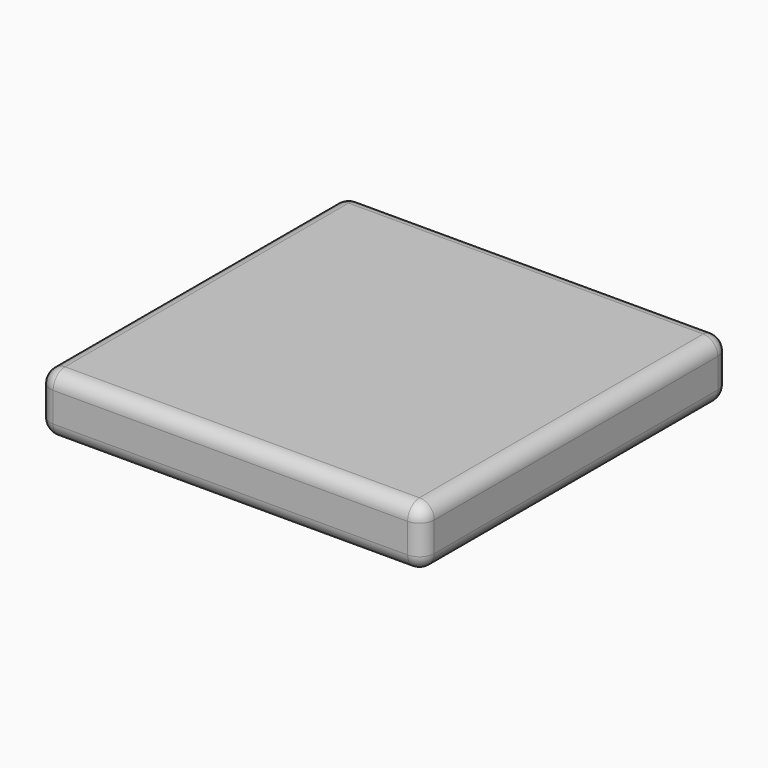
from build123d import *

# Parameters (mm, degrees)
F0_W         = 520
F0_H         = 520
F1_DEPTH     = 80
F2_R         = 20
F3_T1_DEPTH  = 40
F3_S5_W      = 20
F3_S5_H      = 20
F3_T6_DEPTH  = 20
F3_S11_W     = 20
F3_S11_H     = 20
F3_T12_DEPTH = 20
F3_S17_W     = 20
F3_S17_H     = 20
F3_T18_DEPTH = 20
F3_S23_W     = 20
F3_S23_H     = 20
F3_T24_DEPTH = 20
F3_S29_W     = 20
F3_S29_H     = 20
F3_T30_DEPTH = 20
F3_S35_W     = 20
F3_S35_H     = 20
F3_T36_DEPTH = 20
F3_S41_W     = 20
F3_S41_H     = 20
F3_T42_DEPTH = 20
F3_S47_W     = 20
F3_S47_H     = 20
F3_T48_DEPTH = 20


# Not quite as in the source:
# - a fillet or chamfer that OpenCascade refuses, or shapes differently, is made with other operations: its cross-section is extruded or revolved along the edge and cut away or added


with BuildPart() as f1:
    # F0 (on Top) → F1 (new body)
    with BuildSketch(Plane.XY):
        Rectangle(F0_W, F0_H)
    extrude(amount=F1_DEPTH)

    # F2
    f2_edges = [f1.edges().sort_by_distance(p)[0] for p in [
        (260, 0, 80),
        (0, 260, 80),
        (-260, 0, 80),
        (0, -260, 80),
        (0, -260, 0),
        (260, 0, 0),
        (0, 260, 0),
        (-260, 0, 0),
    ]]
    fillet(f2_edges, radius=F2_R)

    # F3: fillet of radius 20 on 4 edges, made by hand

    # F3_s2 → F3_t1 (cut)
    with BuildSketch(Plane.XY.offset(20)):
        with BuildLine():
            ThreePointArc((240, -260), (254.1421356237, -254.1421356237), (260, -240))
            Line((260, -240), (260, -260))
            Line((260, -260), (240, -260))
        make_face()
        with BuildLine():
            ThreePointArc((260, 240), (254.1421356237, 254.1421356237), (240, 260))
            Line((240, 260), (260, 260))
            Line((260, 260), (260, 240))
        make_face()
        with BuildLine():
            ThreePointArc((-260, 240), (-254.1421356237, 254.1421356237), (-240, 260))
            Line((-240, 260), (-260, 260))
            Line((-260, 260), (-260, 240))
        make_face()
        with BuildLine():
            ThreePointArc((-240, -260), (-254.1421356237, -254.1421356237), (-260, -240))
            Line((-260, -240), (-260, -260))
            Line((-260, -260), (-240, -260))
        make_face()
    extrude(amount=F3_T1_DEPTH, mode=Mode.SUBTRACT)


with BuildPart() as f3_tool4:
    # F3_s5 → F3_t6 (new body)
    with BuildSketch(Plane.XZ.offset(240)):
        with Locations((-250, 10)):
            Rectangle(F3_S5_W, F3_S5_H)
    extrude(amount=F3_T6_DEPTH)

    # F3_s7 → F3_t8 (revolve, cut)
    with BuildSketch(Plane(origin=(-240, -240, 20), x_dir=(0.7071067812, 0, 0.7071067812), z_dir=(0.7071067812, 0, -0.7071067812))):
        with BuildLine():
            ThreePointArc((0, -20), (20, 0), (0, 20))
            Line((0, 20), (0, -20))
        make_face()
    revolve(axis=Axis((-240, -240, 20), (0, -1, 0)), mode=Mode.SUBTRACT)


with BuildPart() as f1_1:
    add(f1.part)

    # F3_t3: cut F3_tool4
    add(f3_tool4.part, mode=Mode.SUBTRACT)


with BuildPart() as f3_tool10:
    # F3_s11 → F3_t12 (new body)
    with BuildSketch(Plane.XZ.offset(240)):
        with Locations((-250, 70)):
            Rectangle(F3_S11_W, F3_S11_H)
    extrude(amount=F3_T12_DEPTH)

    # F3_s13 → F3_t14 (revolve, cut)
    with BuildSketch(Plane(origin=(-240, -240, 60), x_dir=(0.7071067812, 0, -0.7071067812), z_dir=(-0.7071067812, 0, -0.7071067812))):
        with BuildLine():
            ThreePointArc((0, -20), (20, 0), (0, 20))
            Line((0, 20), (0, -20))
        make_face()
    revolve(axis=Axis((-240, -240, 60), (0, -1, 0)), mode=Mode.SUBTRACT)


with BuildPart() as f1_2:
    add(f1_1.part)

    # F3_t9: cut F3_tool10
    add(f3_tool10.part, mode=Mode.SUBTRACT)


with BuildPart() as f3_tool16:
    # F3_s17 → F3_t18 (new body)
    with BuildSketch(Plane.YZ.offset(-240)):
        with Locations((250, 10)):
            Rectangle(F3_S17_W, F3_S17_H)
    extrude(amount=-F3_T18_DEPTH)

    # F3_s19 → F3_t20 (revolve, cut)
    with BuildSketch(Plane(origin=(-240, 240, 20), x_dir=(0, -0.7071067812, 0.7071067812), z_dir=(0, -0.7071067812, -0.7071067812))):
        with BuildLine():
            ThreePointArc((0, -20), (20, 0), (0, 20))
            Line((0, 20), (0, -20))
        make_face()
    revolve(axis=Axis((-240, 240, 20), (-1, 0, 0)), mode=Mode.SUBTRACT)


with BuildPart() as f1_3:
    add(f1_2.part)

    # F3_t15: cut F3_tool16
    add(f3_tool16.part, mode=Mode.SUBTRACT)


with BuildPart() as f3_tool22:
    # F3_s23 → F3_t24 (new body)
    with BuildSketch(Plane.YZ.offset(-240)):
        with Locations((250, 70)):
            Rectangle(F3_S23_W, F3_S23_H)
    extrude(amount=-F3_T24_DEPTH)

    # F3_s25 → F3_t26 (revolve, cut)
    with BuildSketch(Plane(origin=(-240, 240, 60), x_dir=(0, -0.7071067812, -0.7071067812), z_dir=(0, 0.7071067812, -0.7071067812))):
        with BuildLine():
            ThreePointArc((0, -20), (20, 0), (0, 20))
            Line((0, 20), (0, -20))
        make_face()
    revolve(axis=Axis((-240, 240, 60), (-1, 0, 0)), mode=Mode.SUBTRACT)


with BuildPart() as f1_4:
    add(f1_3.part)

    # F3_t21: cut F3_tool22
    add(f3_tool22.part, mode=Mode.SUBTRACT)


with BuildPart() as f3_tool28:
    # F3_s29 → F3_t30 (new body)
    with BuildSketch(Plane.YZ.offset(240)):
        with Locations((250, 10)):
            Rectangle(F3_S29_W, F3_S29_H)
    extrude(amount=F3_T30_DEPTH)

    # F3_s31 → F3_t32 (revolve, cut)
    with BuildSketch(Plane(origin=(240, 240, 20), x_dir=(0, -0.7071067812, 0.7071067812), z_dir=(0, 0.7071067812, 0.7071067812))):
        with BuildLine():
            ThreePointArc((0, -20), (20, 0), (0, 20))
            Line((0, 20), (0, -20))
        make_face()
    revolve(axis=Axis((240, 240, 20), (1, 0, 0)), mode=Mode.SUBTRACT)


with BuildPart() as f1_5:
    add(f1_4.part)

    # F3_t27: cut F3_tool28
    add(f3_tool28.part, mode=Mode.SUBTRACT)


with BuildPart() as f3_tool34:
    # F3_s35 → F3_t36 (new body)
    with BuildSketch(Plane.YZ.offset(240)):
        with Locations((250, 70)):
            Rectangle(F3_S35_W, F3_S35_H)
    extrude(amount=F3_T36_DEPTH)

    # F3_s37 → F3_t38 (revolve, cut)
    with BuildSketch(Plane(origin=(240, 240, 60), x_dir=(0, -0.7071067812, -0.7071067812), z_dir=(0, -0.7071067812, 0.7071067812))):
        with BuildLine():
            ThreePointArc((0, -20), (20, 0), (0, 20))
            Line((0, 20), (0, -20))
        make_face()
    revolve(axis=Axis((240, 240, 60), (1, 0, 0)), mode=Mode.SUBTRACT)


with BuildPart() as f1_6:
    add(f1_5.part)

    # F3_t33: cut F3_tool34
    add(f3_tool34.part, mode=Mode.SUBTRACT)


with BuildPart() as f3_tool40:
    # F3_s41 → F3_t42 (new body)
    with BuildSketch(Plane.XZ.offset(240)):
        with Locations((250, 10)):
            Rectangle(F3_S41_W, F3_S41_H)
    extrude(amount=F3_T42_DEPTH)

    # F3_s43 → F3_t44 (revolve, cut)
    with BuildSketch(Plane(origin=(240, -240, 20), x_dir=(-0.7071067812, 0, 0.7071067812), z_dir=(0.7071067812, 0, 0.7071067812))):
        with BuildLine():
            ThreePointArc((0, -20), (20, 0), (0, 20))
            Line((0, 20), (0, -20))
        make_face()
    revolve(axis=Axis((240, -240, 20), (0, -1, 0)), mode=Mode.SUBTRACT)


with BuildPart() as f1_7:
    add(f1_6.part)

    # F3_t39: cut F3_tool40
    add(f3_tool40.part, mode=Mode.SUBTRACT)


with BuildPart() as f3_tool46:
    # F3_s47 → F3_t48 (new body)
    with BuildSketch(Plane.XZ.offset(240)):
        with Locations((250, 70)):
            Rectangle(F3_S47_W, F3_S47_H)
    extrude(amount=F3_T48_DEPTH)

    # F3_s49 → F3_t50 (revolve, cut)
    with BuildSketch(Plane(origin=(240, -240, 60), x_dir=(-0.7071067812, 0, -0.7071067812), z_dir=(-0.7071067812, 0, 0.7071067812))):
        with BuildLine():
            ThreePointArc((0, -20), (20, 0), (0, 20))
            Line((0, 20), (0, -20))
        make_face()
    revolve(axis=Axis((240, -240, 60), (0, -1, 0)), mode=Mode.SUBTRACT)


with BuildPart() as f1_8:
    add(f1_7.part)

    # F3_t45: cut F3_tool46
    add(f3_tool46.part, mode=Mode.SUBTRACT)


solid = f1_8.part
